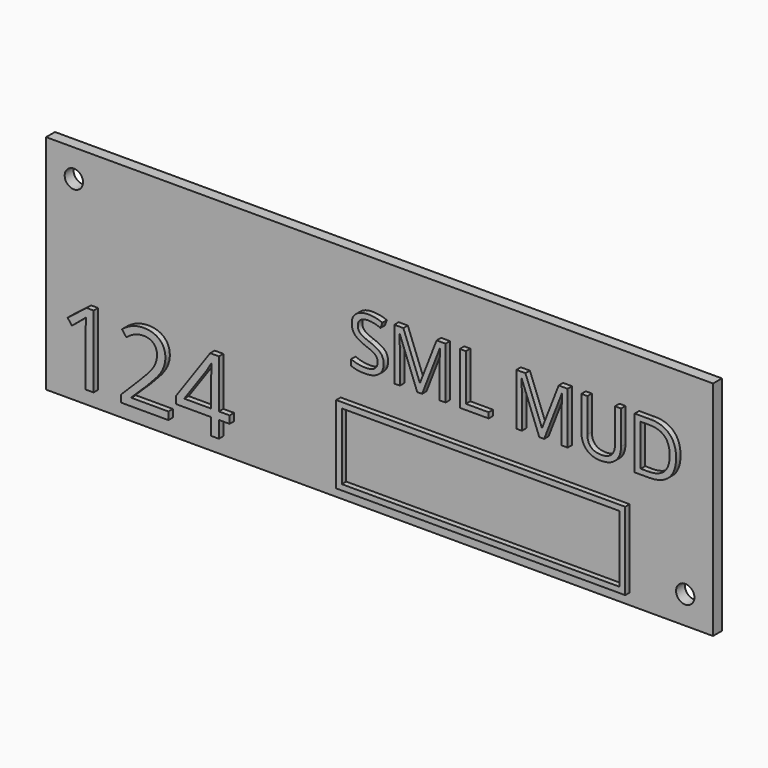
from build123d import *

# Parameters (mm, degrees)
F0_W         = 120
F0_H         = 40
F1_DEPTH     = 2
F3_D         = 3.3
F4_TEXT_SIZE = 13.0598918478
F5_DEPTH     = 1
F6_TEXT_SIZE = 18.1818181818
F7_DEPTH     = 1
F8_W         = 52
F8_H         = 14
F8_W_2       = 49.99999962
F8_H_2       = 11.99999962
F9_DEPTH     = 1


# Not quite as in the source:
# - Text() gives the source's letters only with a copy of the font that has no kerning and outlines rounded to 1/6400 em; it was checked with that copy


with BuildPart() as f1:
    # F0 (on Front) → F1 (new body)
    with BuildSketch(Plane.XZ):
        Rectangle(F0_W, F0_H)
    extrude(amount=F1_DEPTH)

    # F3 (through all)
    with Locations(Plane.XZ.offset(2)):
        with Locations((-55, 15), (55, -15)):
            Hole(F3_D / 2)

    # F4 (on face) → F5 (join)
    with BuildSketch(Plane.XZ.offset(2)):
        with Locations((-5, 2)):
            Text('SML MUD', F4_TEXT_SIZE, font='Open Sans', text_align=(TextAlign.LEFT, TextAlign.BOTTOM))
    extrude(amount=F5_DEPTH)

    # F6 (on face) → F7 (join)
    with BuildSketch(Plane.XZ.offset(2)):
        with Locations((-57, -17)):
            Text('124', F6_TEXT_SIZE, font='Open Sans', text_align=(TextAlign.LEFT, TextAlign.BOTTOM))
    extrude(amount=F7_DEPTH)

    # F8 (on face) → F9 (join)
    with BuildSketch(Plane.XZ.offset(2)):
        with Locations((19, -11)):
            Rectangle(F8_W, F8_H)
        with Locations((19, -11)):
            Rectangle(F8_W_2, F8_H_2, mode=Mode.SUBTRACT)
    extrude(amount=F9_DEPTH)


solid = f1.part
